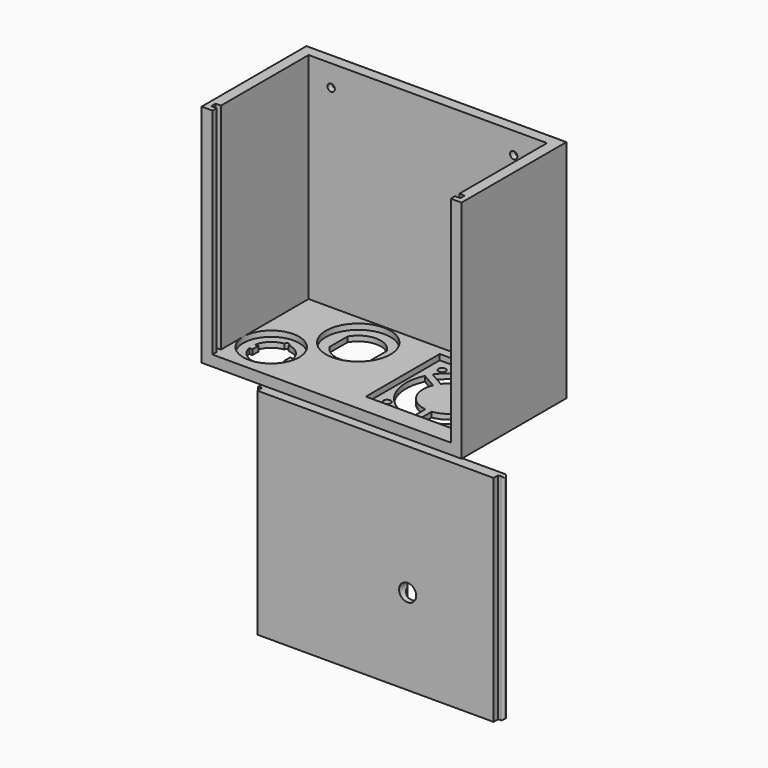
from build123d import *

# Parameters (mm, degrees)
F0_W          = 121
F0_H          = 61
F0_W_2        = 111
F0_H_2        = 51
F1_DEPTH      = 100
F2_W          = 121
F2_H          = 61
F3_DEPTH      = 5
F5_DEPTH      = 25
F7_R          = 1.7
F8_DEPTH      = 25
F10_R         = 1.7
F11_DEPTH     = 25
F12_R         = 3
F13_DEPTH     = 2.2
F14_R         = 15
F14_R_2       = 13
F14_W         = 43
F14_H         = 43
F15_DEPTH     = 2.6
F17_W         = 111
F17_H         = 100
F18_DEPTH     = 25
F20_W         = 2.5
F20_H         = 2.5
F21_DEPTH     = 100
F22_W         = 110
F22_H         = 100
F22_R         = 4
F23_DEPTH     = 5
F24_W         = 2.3
F24_H         = 2.3
F25_DEPTH     = 100
F26_R         = 1
F28_W         = 8
F28_H         = 2.6
F29_DEPTH     = 40.001
F30_T4_DEPTH  = 46.5
F30_S5_R      = 4
F30_T6_DEPTH  = 25
F30_T10_DEPTH = 46.501
F30_S11_R     = 4
F30_T12_DEPTH = 25


# Not quite as in the source:
# - a fillet or chamfer that OpenCascade refuses, or shapes differently, is made with other operations: its cross-section is extruded or revolved along the edge and cut away or added


with BuildPart() as f1:
    # F0 (on Top) → F1 (new body)
    with BuildSketch(Plane.XY):
        Rectangle(F0_W, F0_H)
        Rectangle(F0_W_2, F0_H_2, mode=Mode.SUBTRACT)
    extrude(amount=F1_DEPTH)

    # F2 (on Top) → F3 (join)
    with BuildSketch(Plane.XY):
        Rectangle(F2_W, F2_H)
    extrude(amount=-F3_DEPTH)

    # F4 (on Top) → F5 (cut)
    with BuildSketch(Plane.XY):
        with BuildLine():
            Line((-35.15, -10.75), (-33.6717782085, -10.75))
            ThreePointArc((-33.6717782085, -10.75), (-36.410590764, -5.8728516572), (-41.5015444025, -3.5555555556))
            ThreePointArc((-41.5015444025, -3.5555555556), (-42.5, -2.5), (-43.4984555975, -3.5555555556))
            ThreePointArc((-43.4984555975, -3.5555555556), (-48.589409236, -5.8728516572), (-51.3282217915, -10.75))
            Line((-51.3282217915, -10.75), (-49.85, -10.75))
            Line((-49.85, -10.75), (-49.85, -14.25))
            Line((-49.85, -14.25), (-51.3282217915, -14.25))
            ThreePointArc((-51.3282217915, -14.25), (-42.5, -21.5), (-33.6717782085, -14.25))
            Line((-33.6717782085, -14.25), (-35.15, -14.25))
            Line((-35.15, -14.25), (-35.15, -10.75))
        make_face()
        with BuildLine():
            Line((-29.15, 15.150485414), (-29.15, 4.849514586))
            ThreePointArc((-29.15, 4.849514586), (-20, -0.5), (-10.85, 4.849514586))
            Line((-10.85, 4.849514586), (-10.85, 15.150485414))
            ThreePointArc((-10.85, 15.150485414), (-20, 20.5), (-29.15, 15.150485414))
        make_face()
    extrude(amount=-F5_DEPTH, mode=Mode.SUBTRACT)

    # F7 (on offset) → F8 (cut)
    with BuildSketch(Plane(origin=(0, 30.5, 0), x_dir=(-1, 0, 0), z_dir=(0, 1, 0))):
        with Locations((-40, 90)):
            Circle(F7_R)
        with Locations((45, 90)):
            Circle(F7_R)
    extrude(amount=-F8_DEPTH, mode=Mode.SUBTRACT)

    # F10 (on offset) → F11 (cut)
    with BuildSketch(Plane(origin=(0, 0, -5), x_dir=(1, 0, 0), z_dir=(0, 0, -1))):
        with Locations((14.25, 16)):
            Circle(F10_R)
        with BuildLine():
            Line((28.75, 11.9058808998), (28.75, 19.9436706752))
            ThreePointArc((28.75, 19.9436706752), (12.9572093402, 10.0478550546), (12.1805876672, -8.5730005218))
            Line((12.1805876672, -8.5730005218), (19.1636367266, -4.5926625579))
            ThreePointArc((19.1636367266, -4.5926625579), (19.8743256041, 6.0287130328), (28.75, 11.9058808998))
        make_face()
        with BuildLine():
            Line((31.75, 19.9436706752), (31.75, 11.9058808998))
            ThreePointArc((31.75, 11.9058808998), (40.6256743959, 6.0287130328), (41.3363632734, -4.5926625579))
            Line((41.3363632734, -4.5926625579), (48.3194123328, -8.5730005218))
            ThreePointArc((48.3194123328, -8.5730005218), (47.5427906598, 10.0478550546), (31.75, 19.9436706752))
        make_face()
        with Locations((46.25, 16)):
            Circle(F10_R)
        with BuildLine():
            Line((46.8338032008, -11.1793323324), (39.8507541413, -7.1989943685))
            ThreePointArc((39.8507541413, -7.1989943685), (30.25, -12), (20.6492458587, -7.1989943685))
            Line((20.6492458587, -7.1989943685), (13.6661967992, -11.1793323324))
            ThreePointArc((13.6661967992, -11.1793323324), (30.25, -20), (46.8338032008, -11.1793323324))
        make_face()
        with Locations((14.25, -16)):
            Circle(F10_R)
        with Locations((46.25, -16)):
            Circle(F10_R)
    extrude(amount=-F11_DEPTH, mode=Mode.SUBTRACT)

    # F12 (on offset) → F13 (cut)
    with BuildSketch(Plane(origin=(0, 30.5, 0), x_dir=(-1, 0, 0), z_dir=(0, 1, 0))):
        with Locations((-40, 90)):
            Circle(F12_R)
        with Locations((45, 90)):
            Circle(F12_R)
    extrude(amount=-F13_DEPTH, mode=Mode.SUBTRACT)

    # F14 (on Top) → F15 (cut)
    with BuildSketch(Plane.XY):
        with Locations((-20, 10)):
            Circle(F14_R)
        with Locations((-42.5, -12.5)):
            Circle(F14_R_2)
        with Locations((30.25, 0)):
            Rectangle(F14_W, F14_H)
    extrude(amount=-F15_DEPTH, mode=Mode.SUBTRACT)

    # F17 (on offset) → F18 (cut)
    with BuildSketch(Plane.XZ.offset(30.5)):
        with Locations((0, 50)):
            Rectangle(F17_W, F17_H)
    extrude(amount=-F18_DEPTH, mode=Mode.SUBTRACT)

    # F20 (on offset) → F21 (cut)
    with BuildSketch(Plane.XY.offset(100)):
        with Locations((-56.75, -26.75)):
            Rectangle(F20_W, F20_H)
        with Locations((56.75, -26.75)):
            Rectangle(F20_W, F20_H)
    extrude(amount=-F21_DEPTH, mode=Mode.SUBTRACT)


with BuildPart() as f23:
    # F22 (on Front) → F23 (new body)
    with BuildSketch(Plane.XZ):
        with Locations((0, -75)):
            Rectangle(F22_W, F22_H)
        with Locations((15, -85)):
            Circle(F22_R, mode=Mode.SUBTRACT)
    extrude(amount=F23_DEPTH)

    # F24 (on face) → F25 (join)
    with BuildSketch(Plane(origin=(0, 0, -125), x_dir=(1, 0, 0), z_dir=(0, 0, -1))):
        with Locations((56.15, 1.15)):
            Rectangle(F24_W, F24_H)
        with Locations((-56.15, 1.15)):
            Rectangle(F24_W, F24_H)
    extrude(amount=-F25_DEPTH)

    # F26
    f26_edges = [f23.edges().sort_by_distance(p)[0] for p in [
        (57.3, 0, -75),
        (57.3, -2.3, -75),
        (57.3, -1.15, -125),
        (57.3, -1.15, -25),
        (-57.3, -2.3, -75),
        (-57.3, 0, -75),
        (-57.3, -1.15, -125),
        (-57.3, -1.15, -25),
    ]]
    fillet(f26_edges, radius=F26_R)

    # F28 (on offset) → F29 (cut, through all)
    with BuildSketch(Plane(origin=(0, 0, -125), x_dir=(1, 0, 0), z_dir=(0, 0, -1))):
        with Locations((15, 1.3)):
            Rectangle(F28_W, F28_H)
    extrude(amount=-F29_DEPTH, mode=Mode.SUBTRACT)

    # F30: fillet of radius 2.6 on 2 edges, made by hand


with BuildPart() as f30_tool2:
    # F30_s3 → F30_t4 (new body)
    with BuildSketch(Plane.XY.offset(-125)):
        with BuildLine():
            ThreePointArc((19, 0), (18.2384776311, -1.8384776311), (16.4, -2.6))
            Line((16.4, -2.6), (19, -2.6))
            Line((19, -2.6), (19, 0))
        make_face()
    extrude(amount=F30_T4_DEPTH)

    # F30_s5 → F30_t6 (cut, symmetric)
    with BuildSketch(Plane.XZ.offset(1.3)):
        with Locations((15, -85)):
            Circle(F30_S5_R)
    extrude(amount=F30_T6_DEPTH, both=True, mode=Mode.SUBTRACT)


with BuildPart() as f23_1:
    add(f23.part)

    # F30_t1: union F30_tool2
    add(f30_tool2.part)


with BuildPart() as f30_tool8:
    # F30_s9 → F30_t10 (new body)
    with BuildSketch(Plane.XY.offset(-125)):
        with BuildLine():
            ThreePointArc((13.6, -2.6), (11.7615223689, -1.8384776311), (11, 0))
            Line((11, 0), (11, -2.6))
            Line((11, -2.6), (13.6, -2.6))
        make_face()
    extrude(amount=F30_T10_DEPTH)

    # F30_s11 → F30_t12 (cut, symmetric)
    with BuildSketch(Plane.XZ.offset(1.3)):
        with Locations((15, -85)):
            Circle(F30_S11_R)
    extrude(amount=F30_T12_DEPTH, both=True, mode=Mode.SUBTRACT)


with BuildPart() as f23_2:
    add(f23_1.part)

    # F30_t7: union F30_tool8
    add(f30_tool8.part)


solid = Compound([f1.part, f23_2.part])
